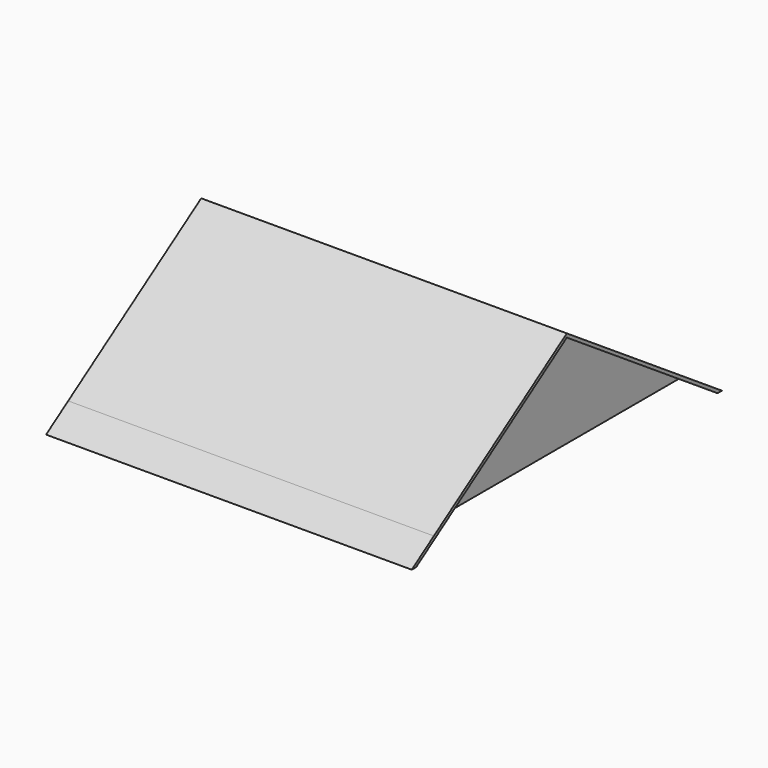
from build123d import *

# Parameters (mm, degrees)
F0_W     = 152.4
F0_H     = 152.4
F1_DEPTH = 50.8
F3_DEPTH = 152.401
F5_DEPTH = 7.62
F7_DEPTH = 7.62
F9_DEPTH = 167.64


with BuildPart() as f1:
    # F0 (on Top) → F1 (new body)
    with BuildSketch(Plane.XY):
        Rectangle(F0_W, F0_H)
    extrude(amount=F1_DEPTH)

    # F2 (on face) → F3 (cut, through all)
    with BuildSketch(Plane(origin=(-76.2, 0, 0), x_dir=(0, -1, 0), z_dir=(-1, 0, 0))):
        Polygon((76.2, 50.8), (0, 50.8), (76.2, 0), align=None)
        Polygon((-76.2, 0), (0, 50.8), (-76.2, 50.8), align=None)
    extrude(amount=-F3_DEPTH, mode=Mode.SUBTRACT)

    # F4 (on face) → F5 (join)
    with BuildSketch(Plane.YZ.offset(76.2)):
        Polygon((-76.2, 0), (-73.66, 0), (0, 49.1066666667), (73.66, 0), (76.2, 0), (0, 50.8), align=None)
    extrude(amount=F5_DEPTH)

    # F6 (on face) → F7 (join)
    with BuildSketch(Plane(origin=(-76.2, 0, 0), x_dir=(0, -1, 0), z_dir=(-1, 0, 0))):
        Polygon((-76.2, 0), (-73.66, 0), (0, 49.0982), (73.66, 0), (76.2, 0), (0, 50.8), align=None)
    extrude(amount=F7_DEPTH)

    # F8 (on face) → F9 (join)
    with BuildSketch(Plane.YZ.offset(83.82)):
        Polygon((-86.3404464857, -8.4536309905), (-73.66, 0), (-76.2, 0), (-88.8804464857, -8.4536309905), align=None)
        Polygon((76.2, 0), (73.66, 0), (86.3404464857, -8.4536309905), (88.8804464857, -8.4536309905), align=None)
    extrude(amount=-F9_DEPTH)


solid = f1.part
